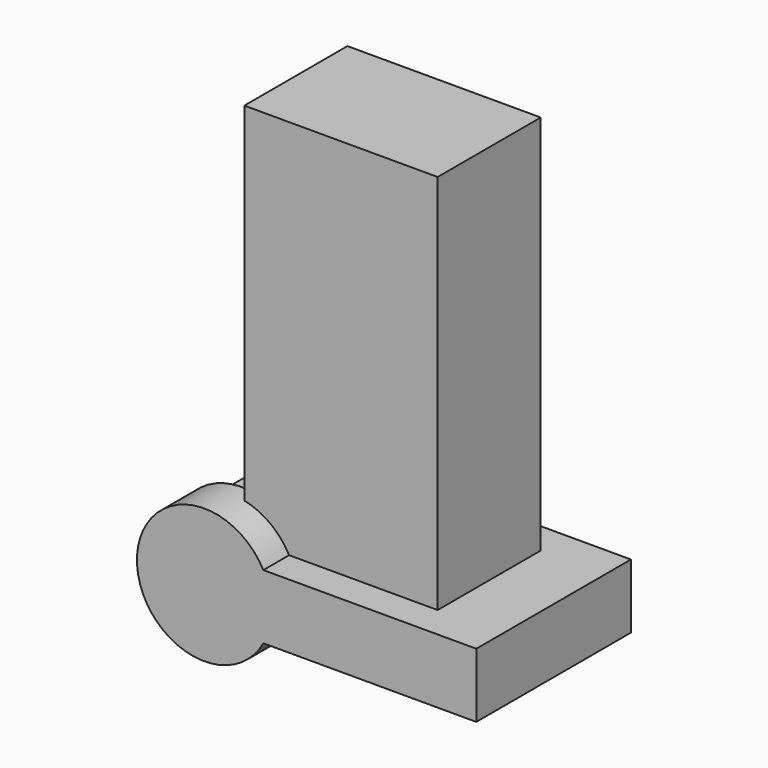
from build123d import *

# Parameters (mm, degrees)
F0_W     = 63.5
F0_H     = 38.1
F1_DEPTH = 6.35
F2_W     = 38.1
F2_H     = 25.4
F3_DEPTH = 75.1442132
F5_DEPTH = 9.144


# Not quite as in the source:
# - an extrude ends at something that could not be found from the text; its depth is read off the source's solid


with BuildPart() as f1:
    # F0 (on Top) → F1 (new body, symmetric)
    with BuildSketch(Plane.XY):
        Rectangle(F0_W, F0_H)
    extrude(amount=F1_DEPTH, both=True)

    # F2 (on face) → F3 (join, through all)
    with BuildSketch(Plane.XY.offset(6.35)):
        Rectangle(F2_W, F2_H)
    extrude(amount=F3_DEPTH)

    # F4 (on face) → F5 (join)
    with BuildSketch(Plane.XZ.offset(19.05)):
        with BuildLine():
            Line((-31.75, 6.35), (-10.2243826786, 6.35))
            ThreePointArc((-10.2243826786, 6.35), (-35.1404271759, 0), (-10.2243826786, -6.35))
            Line((-10.2243826786, -6.35), (-31.75, -6.35))
            Line((-31.75, -6.35), (-31.75, 6.35))
        make_face()
    extrude(amount=-F5_DEPTH)


solid = f1.part
